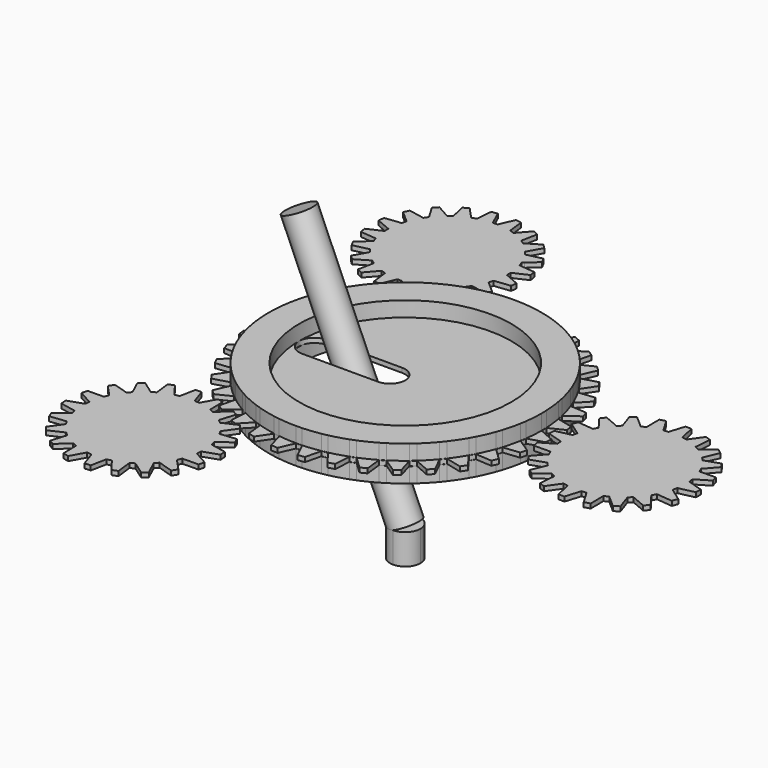
from build123d import *

# Parameters (mm, degrees)
F1_DEPTH  = 3
F2_DEPTH  = 3
F3_DEPTH  = 3
F4_DEPTH  = 3
F5_START  = 3.1
F5_DEPTH  = 10
F11_DEPTH = 20
F15_R     = 10


with BuildPart() as f1:
    # F0 (on Top) → F1 (new body)
    with BuildSketch(Plane.XY):
        with BuildLine():
            ThreePointArc((89.2300375236, -11.7473572998), (89.8073030915, -5.8862816307), (90, 0))
            Line((90, 0), (89.9143399424, 3.9257448629))
            ThreePointArc((89.9143399424, 3.9257448629), (89.46507044, 9.7980187367), (88.6326977711, 15.62833599))
            Line((88.6326977711, 15.62833599), (87.8666406408, 19.4795652544))
            ThreePointArc((87.8666406408, 19.4795652544), (86.4044868947, 25.1846112628), (84.5723358707, 30.7818128993))
            Line((84.5723358707, 30.7818128993), (83.149157926, 34.4415089129))
            ThreePointArc((83.149157926, 34.4415089129), (80.7185467379, 39.8059821197), (77.9422863406, 45))
            Line((77.9422863406, 45), (75.9052301232, 48.3569647512))
            ThreePointArc((75.9052301232, 48.3569647512), (72.5800143841, 53.2178683527), (68.9439998807, 57.8508848718))
            Line((68.9439998807, 57.8508848718), (66.3549603129, 60.8031186854))
            ThreePointArc((66.3549603129, 60.8031186854), (62.2361750204, 65.0127565854), (57.8508848718, 68.9439998807))
            Line((57.8508848718, 68.9439998807), (54.7885286108, 71.4018006262))
            ThreePointArc((54.7885286108, 71.4018006262), (50.0013209718, 74.8322651072), (45, 77.9422863406))
            Line((45, 77.9422863406), (41.5573751912, 79.830974986))
            ThreePointArc((41.5573751912, 79.830974986), (36.2472020873, 82.3780331208), (30.7818128993, 84.5723358707))
            Line((30.7818128993, 84.5723358707), (27.0635219554, 85.8345255673))
            ThreePointArc((27.0635219554, 85.8345255673), (21.3917303094, 87.4207862832), (15.62833599, 88.6326977711))
            Line((15.62833599, 88.6326977711), (11.7473572998, 89.2300375236))
            ThreePointArc((11.7473572998, 89.2300375236), (5.8862816307, 89.8073030915), (0, 90))
            Line((0, 90), (-3.9257448629, 89.9143399424))
            ThreePointArc((-3.9257448629, 89.9143399424), (-9.7980187367, 89.46507044), (-15.62833599, 88.6326977711))
            Line((-15.62833599, 88.6326977711), (-19.4795652544, 87.8666406408))
            ThreePointArc((-19.4795652544, 87.8666406408), (-25.1846112628, 86.4044868947), (-30.7818128993, 84.5723358707))
            Line((-30.7818128993, 84.5723358707), (-34.4415089129, 83.149157926))
            ThreePointArc((-34.4415089129, 83.149157926), (-39.8059821197, 80.7185467379), (-45, 77.9422863406))
            Line((-45, 77.9422863406), (-48.3569647512, 75.9052301232))
            ThreePointArc((-48.3569647512, 75.9052301232), (-53.2178683527, 72.5800143841), (-57.8508848718, 68.9439998807))
            Line((-57.8508848718, 68.9439998807), (-60.8031186854, 66.3549603129))
            ThreePointArc((-60.8031186854, 66.3549603129), (-65.0127565854, 62.2361750204), (-68.9439998807, 57.8508848718))
            Line((-68.9439998807, 57.8508848718), (-71.4018006262, 54.7885286108))
            ThreePointArc((-71.4018006262, 54.7885286108), (-74.8322651072, 50.0013209718), (-77.9422863406, 45))
            Line((-77.9422863406, 45), (-79.830974986, 41.5573751912))
            ThreePointArc((-79.830974986, 41.5573751912), (-82.3780331208, 36.2472020873), (-84.5723358707, 30.7818128993))
            Line((-84.5723358707, 30.7818128993), (-85.8345255673, 27.0635219554))
            ThreePointArc((-85.8345255673, 27.0635219554), (-87.4207862832, 21.3917303094), (-88.6326977711, 15.62833599))
            Line((-88.6326977711, 15.62833599), (-89.2300375236, 11.7473572998))
            ThreePointArc((-89.2300375236, 11.7473572998), (-89.8073030915, 5.8862816307), (-90, 0))
            Line((-90, 0), (-89.9143399424, -3.9257448629))
            ThreePointArc((-89.9143399424, -3.9257448629), (-89.46507044, -9.7980187367), (-88.6326977711, -15.62833599))
            Line((-88.6326977711, -15.62833599), (-87.8666406408, -19.4795652544))
            ThreePointArc((-87.8666406408, -19.4795652544), (-86.4044868947, -25.1846112628), (-84.5723358707, -30.7818128993))
            Line((-84.5723358707, -30.7818128993), (-83.149157926, -34.4415089129))
            ThreePointArc((-83.149157926, -34.4415089129), (-80.7185467379, -39.8059821197), (-77.9422863406, -45))
            Line((-77.9422863406, -45), (-75.9052301232, -48.3569647512))
            ThreePointArc((-75.9052301232, -48.3569647512), (-72.5800143841, -53.2178683527), (-68.9439998807, -57.8508848718))
            Line((-68.9439998807, -57.8508848718), (-66.3549603129, -60.8031186854))
            ThreePointArc((-66.3549603129, -60.8031186854), (-62.2361750204, -65.0127565854), (-57.8508848718, -68.9439998807))
            Line((-57.8508848718, -68.9439998807), (-54.7885286108, -71.4018006262))
            ThreePointArc((-54.7885286108, -71.4018006262), (-50.0013209718, -74.8322651072), (-45, -77.9422863406))
            Line((-45, -77.9422863406), (-41.5573751912, -79.830974986))
            ThreePointArc((-41.5573751912, -79.830974986), (-36.2472020873, -82.3780331208), (-30.7818128993, -84.5723358707))
            Line((-30.7818128993, -84.5723358707), (-27.0635219554, -85.8345255673))
            ThreePointArc((-27.0635219554, -85.8345255673), (-21.3917303094, -87.4207862832), (-15.62833599, -88.6326977711))
            Line((-15.62833599, -88.6326977711), (-11.7473572998, -89.2300375236))
            ThreePointArc((-11.7473572998, -89.2300375236), (-5.8862816307, -89.8073030915), (0, -90))
            Line((0, -90), (3.9257448629, -89.9143399424))
            ThreePointArc((3.9257448629, -89.9143399424), (9.7980187367, -89.46507044), (15.62833599, -88.6326977711))
            Line((15.62833599, -88.6326977711), (19.4795652544, -87.8666406408))
            ThreePointArc((19.4795652544, -87.8666406408), (25.1846112628, -86.4044868947), (30.7818128993, -84.5723358707))
            Line((30.7818128993, -84.5723358707), (34.4415089129, -83.149157926))
            ThreePointArc((34.4415089129, -83.149157926), (39.8059821197, -80.7185467379), (45, -77.9422863406))
            Line((45, -77.9422863406), (48.3569647512, -75.9052301232))
            ThreePointArc((48.3569647512, -75.9052301232), (53.2178683527, -72.5800143841), (57.8508848718, -68.9439998807))
            Line((57.8508848718, -68.9439998807), (60.8031186854, -66.3549603129))
            ThreePointArc((60.8031186854, -66.3549603129), (65.0127565854, -62.2361750204), (68.9439998807, -57.8508848718))
            Line((68.9439998807, -57.8508848718), (71.4018006262, -54.7885286108))
            ThreePointArc((71.4018006262, -54.7885286108), (74.8322651072, -50.0013209718), (77.9422863406, -45))
            Line((77.9422863406, -45), (79.830974986, -41.5573751912))
            ThreePointArc((79.830974986, -41.5573751912), (82.3780331208, -36.2472020873), (84.5723358707, -30.7818128993))
            Line((84.5723358707, -30.7818128993), (85.8345255673, -27.0635219554))
            ThreePointArc((85.8345255673, -27.0635219554), (87.4207862832, -21.3917303094), (88.6326977711, -15.62833599))
            Line((88.6326977711, -15.62833599), (89.2300375236, -11.7473572998))
        make_face()
        with BuildLine():
            ThreePointArc((-70, 0), (0, 70), (70, 0))
            ThreePointArc((70, 0), (0, -70), (-70, 0))
        make_face(mode=Mode.SUBTRACT)
        with BuildLine():
            ThreePointArc((-10, 10), (-2.9289321881, 7.0710678119), (0, 0))
            Line((0, 0), (70, 0))
            ThreePointArc((70, 0), (0, 70), (-70, 0))
            ThreePointArc((-70, 0), (-67.0710678119, 7.0710678119), (-60, 10))
            Line((-60, 10), (-35, 10))
            Line((-35, 10), (-10, 10))
        make_face()
        with BuildLine():
            Line((70, 0), (0, 0))
            ThreePointArc((0, 0), (-2.9289321881, -7.0710678119), (-10, -10))
            Line((-10, -10), (-35, -10))
            Line((-35, -10), (-60, -10))
            ThreePointArc((-60, -10), (-67.0710678119, -7.0710678119), (-70, 0))
            ThreePointArc((-70, 0), (0, -70), (70, 0))
        make_face()
        with BuildLine():
            Line((99.9048221582, -4.3619387365), (90, 0))
            ThreePointArc((90, 0), (89.8073030915, -5.8862816307), (89.2300375236, -11.7473572998))
            Line((89.2300375236, -11.7473572998), (99.6194698092, -8.7155742748))
            Line((99.6194698092, -8.7155742748), (99.9048221582, -4.3619387365))
        make_face()
        with BuildLine():
            ThreePointArc((-45, 77.9422863406), (-39.8059821197, 80.7185467379), (-34.4415089129, 83.149157926))
            Line((-34.4415089129, 83.149157926), (-42.2618261741, 90.6307787037))
            Line((-42.2618261741, 90.6307787037), (-46.1748613235, 88.7010833178))
            Line((-46.1748613235, 88.7010833178), (-45, 77.9422863406))
        make_face()
        with BuildLine():
            ThreePointArc((-57.8508848718, 68.9439998807), (-53.2178683527, 72.5800143841), (-48.3569647512, 75.9052301232))
            Line((-48.3569647512, 75.9052301232), (-57.3576436351, 81.9152044289))
            Line((-57.3576436351, 81.9152044289), (-60.8761429009, 79.3353340291))
            Line((-60.8761429009, 79.3353340291), (-57.8508848718, 68.9439998807))
        make_face()
        with BuildLine():
            ThreePointArc((-68.9439998807, 57.8508848718), (-65.0127565854, 62.2361750204), (-60.8031186854, 66.3549603129))
            Line((-60.8031186854, 66.3549603129), (-70.7106781187, 70.7106781187))
            Line((-70.7106781187, 70.7106781187), (-73.727733681, 67.5590207616))
            Line((-73.727733681, 67.5590207616), (-68.9439998807, 57.8508848718))
        make_face()
        with BuildLine():
            ThreePointArc((-77.9422863406, 45), (-74.8322651072, 50.0013209718), (-71.4018006262, 54.7885286108))
            Line((-71.4018006262, 54.7885286108), (-81.9152044289, 57.3576436351))
            Line((-81.9152044289, 57.3576436351), (-84.3391445813, 53.7299608347))
            Line((-84.3391445813, 53.7299608347), (-77.9422863406, 45))
        make_face()
        with BuildLine():
            ThreePointArc((-84.5723358707, 30.7818128993), (-82.3780331208, 36.2472020873), (-79.830974986, 41.5573751912))
            Line((-79.830974986, 41.5573751912), (-90.6307787037, 42.2618261741))
            Line((-90.6307787037, 42.2618261741), (-92.3879532511, 38.2683432365))
            Line((-92.3879532511, 38.2683432365), (-84.5723358707, 30.7818128993))
        make_face()
        with BuildLine():
            Line((-99.1444861374, -13.052619222), (-88.6326977711, -15.62833599))
            ThreePointArc((-88.6326977711, -15.62833599), (-89.46507044, -9.7980187367), (-89.9143399424, -3.9257448629))
            Line((-89.9143399424, -3.9257448629), (-99.6194698092, -8.7155742748))
            Line((-99.6194698092, -8.7155742748), (-99.1444861374, -13.052619222))
        make_face()
        with BuildLine():
            ThreePointArc((-88.6326977711, 15.62833599), (-87.4207862832, 21.3917303094), (-85.8345255673, 27.0635219554))
            Line((-85.8345255673, 27.0635219554), (-96.5925826289, 25.8819045103))
            Line((-96.5925826289, 25.8819045103), (-97.629600712, 21.6439613938))
            Line((-97.629600712, 21.6439613938), (-88.6326977711, 15.62833599))
        make_face()
        with BuildLine():
            ThreePointArc((-90, 0), (-89.8073030915, 5.8862816307), (-89.2300375236, 11.7473572998))
            Line((-89.2300375236, 11.7473572998), (-99.6194698092, 8.7155742748))
            Line((-99.6194698092, 8.7155742748), (-99.9048221582, 4.3619387365))
            Line((-99.9048221582, 4.3619387365), (-90, 0))
        make_face()
        with BuildLine():
            Line((-88.7010833178, -46.1748613235), (-77.9422863406, -45))
            ThreePointArc((-77.9422863406, -45), (-80.7185467379, -39.8059821197), (-83.149157926, -34.4415089129))
            Line((-83.149157926, -34.4415089129), (-90.6307787037, -42.2618261741))
            Line((-90.6307787037, -42.2618261741), (-88.7010833178, -46.1748613235))
        make_face()
        with BuildLine():
            Line((-79.3353340291, -60.8761429009), (-68.9439998807, -57.8508848718))
            ThreePointArc((-68.9439998807, -57.8508848718), (-72.5800143841, -53.2178683527), (-75.9052301232, -48.3569647512))
            Line((-75.9052301232, -48.3569647512), (-81.9152044289, -57.3576436351))
            Line((-81.9152044289, -57.3576436351), (-79.3353340291, -60.8761429009))
        make_face()
        with BuildLine():
            Line((-95.3716950748, -30.0705799504), (-84.5723358707, -30.7818128993))
            ThreePointArc((-84.5723358707, -30.7818128993), (-86.4044868947, -25.1846112628), (-87.8666406408, -19.4795652544))
            Line((-87.8666406408, -19.4795652544), (-96.5925826289, -25.8819045103))
            Line((-96.5925826289, -25.8819045103), (-95.3716950748, -30.0705799504))
        make_face()
        with BuildLine():
            Line((60.8761429009, -79.3353340291), (57.8508848718, -68.9439998807))
            ThreePointArc((57.8508848718, -68.9439998807), (53.2178683527, -72.5800143841), (48.3569647512, -75.9052301232))
            Line((48.3569647512, -75.9052301232), (57.3576436351, -81.9152044289))
            Line((57.3576436351, -81.9152044289), (60.8761429009, -79.3353340291))
        make_face()
        with BuildLine():
            Line((73.727733681, -67.5590207616), (68.9439998807, -57.8508848718))
            ThreePointArc((68.9439998807, -57.8508848718), (65.0127565854, -62.2361750204), (60.8031186854, -66.3549603129))
            Line((60.8031186854, -66.3549603129), (70.7106781187, -70.7106781187))
            Line((70.7106781187, -70.7106781187), (73.727733681, -67.5590207616))
        make_face()
        with BuildLine():
            Line((84.3391445813, -53.7299608347), (77.9422863406, -45))
            ThreePointArc((77.9422863406, -45), (74.8322651072, -50.0013209718), (71.4018006262, -54.7885286108))
            Line((71.4018006262, -54.7885286108), (81.9152044289, -57.3576436351))
            Line((81.9152044289, -57.3576436351), (84.3391445813, -53.7299608347))
        make_face()
        with BuildLine():
            Line((92.3879532511, -38.2683432365), (84.5723358707, -30.7818128993))
            ThreePointArc((84.5723358707, -30.7818128993), (82.3780331208, -36.2472020873), (79.830974986, -41.5573751912))
            Line((79.830974986, -41.5573751912), (90.6307787037, -42.2618261741))
            Line((90.6307787037, -42.2618261741), (92.3879532511, -38.2683432365))
        make_face()
        with BuildLine():
            Line((30.0705799504, -95.3716950748), (30.7818128993, -84.5723358707))
            ThreePointArc((30.7818128993, -84.5723358707), (25.1846112628, -86.4044868947), (19.4795652544, -87.8666406408))
            Line((19.4795652544, -87.8666406408), (25.8819045103, -96.5925826289))
            Line((25.8819045103, -96.5925826289), (30.0705799504, -95.3716950748))
        make_face()
        with BuildLine():
            Line((46.1748613235, -88.7010833178), (45, -77.9422863406))
            ThreePointArc((45, -77.9422863406), (39.8059821197, -80.7185467379), (34.4415089129, -83.149157926))
            Line((34.4415089129, -83.149157926), (42.2618261741, -90.6307787037))
            Line((42.2618261741, -90.6307787037), (46.1748613235, -88.7010833178))
        make_face()
        with BuildLine():
            Line((13.052619222, -99.1444861374), (15.62833599, -88.6326977711))
            ThreePointArc((15.62833599, -88.6326977711), (9.7980187367, -89.46507044), (3.9257448629, -89.9143399424))
            Line((3.9257448629, -89.9143399424), (8.7155742748, -99.6194698092))
            Line((8.7155742748, -99.6194698092), (13.052619222, -99.1444861374))
        make_face()
        with BuildLine():
            Line((-4.3619387365, -99.9048221582), (0, -90))
            ThreePointArc((0, -90), (-5.8862816307, -89.8073030915), (-11.7473572998, -89.2300375236))
            Line((-11.7473572998, -89.2300375236), (-8.7155742748, -99.6194698092))
            Line((-8.7155742748, -99.6194698092), (-4.3619387365, -99.9048221582))
        make_face()
        with BuildLine():
            Line((-21.6439613938, -97.629600712), (-15.62833599, -88.6326977711))
            ThreePointArc((-15.62833599, -88.6326977711), (-21.3917303094, -87.4207862832), (-27.0635219554, -85.8345255673))
            Line((-27.0635219554, -85.8345255673), (-25.8819045103, -96.5925826289))
            Line((-25.8819045103, -96.5925826289), (-21.6439613938, -97.629600712))
        make_face()
        with BuildLine():
            Line((-38.2683432365, -92.3879532511), (-30.7818128993, -84.5723358707))
            ThreePointArc((-30.7818128993, -84.5723358707), (-36.2472020873, -82.3780331208), (-41.5573751912, -79.830974986))
            Line((-41.5573751912, -79.830974986), (-42.2618261741, -90.6307787037))
            Line((-42.2618261741, -90.6307787037), (-38.2683432365, -92.3879532511))
        make_face()
        with BuildLine():
            Line((-53.7299608347, -84.3391445813), (-45, -77.9422863406))
            ThreePointArc((-45, -77.9422863406), (-50.0013209718, -74.8322651072), (-54.7885286108, -71.4018006262))
            Line((-54.7885286108, -71.4018006262), (-57.3576436351, -81.9152044289))
            Line((-57.3576436351, -81.9152044289), (-53.7299608347, -84.3391445813))
        make_face()
        with BuildLine():
            Line((-67.5590207616, -73.727733681), (-57.8508848718, -68.9439998807))
            ThreePointArc((-57.8508848718, -68.9439998807), (-62.2361750204, -65.0127565854), (-66.3549603129, -60.8031186854))
            Line((-66.3549603129, -60.8031186854), (-70.7106781187, -70.7106781187))
            Line((-70.7106781187, -70.7106781187), (-67.5590207616, -73.727733681))
        make_face()
        with BuildLine():
            Line((97.629600712, -21.6439613938), (88.6326977711, -15.62833599))
            ThreePointArc((88.6326977711, -15.62833599), (87.4207862832, -21.3917303094), (85.8345255673, -27.0635219554))
            Line((85.8345255673, -27.0635219554), (96.5925826289, -25.8819045103))
            Line((96.5925826289, -25.8819045103), (97.629600712, -21.6439613938))
        make_face()
        with BuildLine():
            ThreePointArc((88.6326977711, 15.62833599), (89.46507044, 9.7980187367), (89.9143399424, 3.9257448629))
            Line((89.9143399424, 3.9257448629), (99.6194698092, 8.7155742748))
            Line((99.6194698092, 8.7155742748), (99.1444861374, 13.052619222))
            Line((99.1444861374, 13.052619222), (88.6326977711, 15.62833599))
        make_face()
        with BuildLine():
            ThreePointArc((84.5723358707, 30.7818128993), (86.4044868947, 25.1846112628), (87.8666406408, 19.4795652544))
            Line((87.8666406408, 19.4795652544), (96.5925826289, 25.8819045103))
            Line((96.5925826289, 25.8819045103), (95.3716950748, 30.0705799504))
            Line((95.3716950748, 30.0705799504), (84.5723358707, 30.7818128993))
        make_face()
        with BuildLine():
            ThreePointArc((77.9422863406, 45), (80.7185467379, 39.8059821197), (83.149157926, 34.4415089129))
            Line((83.149157926, 34.4415089129), (90.6307787037, 42.2618261741))
            Line((90.6307787037, 42.2618261741), (88.7010833178, 46.1748613235))
            Line((88.7010833178, 46.1748613235), (77.9422863406, 45))
        make_face()
        with BuildLine():
            ThreePointArc((68.9439998807, 57.8508848718), (72.5800143841, 53.2178683527), (75.9052301232, 48.3569647512))
            Line((75.9052301232, 48.3569647512), (81.9152044289, 57.3576436351))
            Line((81.9152044289, 57.3576436351), (79.3353340291, 60.8761429009))
            Line((79.3353340291, 60.8761429009), (68.9439998807, 57.8508848718))
        make_face()
        with BuildLine():
            ThreePointArc((57.8508848718, 68.9439998807), (62.2361750204, 65.0127565854), (66.3549603129, 60.8031186854))
            Line((66.3549603129, 60.8031186854), (70.7106781187, 70.7106781187))
            Line((70.7106781187, 70.7106781187), (67.5590207616, 73.727733681))
            Line((67.5590207616, 73.727733681), (57.8508848718, 68.9439998807))
        make_face()
        with BuildLine():
            ThreePointArc((45, 77.9422863406), (50.0013209718, 74.8322651072), (54.7885286108, 71.4018006262))
            Line((54.7885286108, 71.4018006262), (57.3576436351, 81.9152044289))
            Line((57.3576436351, 81.9152044289), (53.7299608347, 84.3391445813))
            Line((53.7299608347, 84.3391445813), (45, 77.9422863406))
        make_face()
        with BuildLine():
            ThreePointArc((30.7818128993, 84.5723358707), (36.2472020873, 82.3780331208), (41.5573751912, 79.830974986))
            Line((41.5573751912, 79.830974986), (42.2618261741, 90.6307787037))
            Line((42.2618261741, 90.6307787037), (38.2683432365, 92.3879532511))
            Line((38.2683432365, 92.3879532511), (30.7818128993, 84.5723358707))
        make_face()
        with BuildLine():
            ThreePointArc((-30.7818128993, 84.5723358707), (-25.1846112628, 86.4044868947), (-19.4795652544, 87.8666406408))
            Line((-19.4795652544, 87.8666406408), (-25.8819045103, 96.5925826289))
            Line((-25.8819045103, 96.5925826289), (-30.0705799504, 95.3716950748))
            Line((-30.0705799504, 95.3716950748), (-30.7818128993, 84.5723358707))
        make_face()
        with BuildLine():
            ThreePointArc((-15.62833599, 88.6326977711), (-9.7980187367, 89.46507044), (-3.9257448629, 89.9143399424))
            Line((-3.9257448629, 89.9143399424), (-8.7155742748, 99.6194698092))
            Line((-8.7155742748, 99.6194698092), (-13.052619222, 99.1444861374))
            Line((-13.052619222, 99.1444861374), (-15.62833599, 88.6326977711))
        make_face()
        with BuildLine():
            ThreePointArc((0, 90), (5.8862816307, 89.8073030915), (11.7473572998, 89.2300375236))
            Line((11.7473572998, 89.2300375236), (8.7155742748, 99.6194698092))
            Line((8.7155742748, 99.6194698092), (4.3619387365, 99.9048221582))
            Line((4.3619387365, 99.9048221582), (0, 90))
        make_face()
        with BuildLine():
            ThreePointArc((15.62833599, 88.6326977711), (21.3917303094, 87.4207862832), (27.0635219554, 85.8345255673))
            Line((27.0635219554, 85.8345255673), (25.8819045103, 96.5925826289))
            Line((25.8819045103, 96.5925826289), (21.6439613938, 97.629600712))
            Line((21.6439613938, 97.629600712), (15.62833599, 88.6326977711))
        make_face()
        with BuildLine():
            ThreePointArc((-84.5723358707, -30.7818128993), (-83.8807082355, -32.6194234455), (-83.149157926, -34.4415089129))
            Line((-83.149157926, -34.4415089129), (-84.5723358707, -30.7818128993))
        make_face()
        with BuildLine():
            ThreePointArc((-90, 0), (-89.9785824372, -1.9633396531), (-89.9143399424, -3.9257448629))
            Line((-89.9143399424, -3.9257448629), (-90, 0))
        make_face()
        with BuildLine():
            Line((-85.8345255673, 27.0635219554), (-84.5723358707, 30.7818128993))
            ThreePointArc((-84.5723358707, 30.7818128993), (-85.2237116546, 28.9295518773), (-85.8345255673, 27.0635219554))
        make_face()
        with BuildLine():
            ThreePointArc((-68.9439998807, -57.8508848718), (-67.6655826731, -59.341123359), (-66.3549603129, -60.8031186854))
            Line((-66.3549603129, -60.8031186854), (-68.9439998807, -57.8508848718))
        make_face()
        with BuildLine():
            Line((-89.2300375236, 11.7473572998), (-88.6326977711, 15.62833599))
            ThreePointArc((-88.6326977711, 15.62833599), (-88.9525359421, 13.6911047571), (-89.2300375236, 11.7473572998))
        make_face()
        with BuildLine():
            ThreePointArc((-88.6326977711, -15.62833599), (-88.2706752363, -17.5581289815), (-87.8666406408, -19.4795652544))
            Line((-87.8666406408, -19.4795652544), (-88.6326977711, -15.62833599))
        make_face()
        with BuildLine():
            ThreePointArc((-77.9422863406, -45), (-76.9420683606, -46.6895932344), (-75.9052301232, -48.3569647512))
            Line((-75.9052301232, -48.3569647512), (-77.9422863406, -45))
        make_face()
        with BuildLine():
            Line((-79.830974986, 41.5573751912), (-77.9422863406, 45))
            ThreePointArc((-77.9422863406, 45), (-78.9054080137, 43.2889892027), (-79.830974986, 41.5573751912))
        make_face()
        with BuildLine():
            ThreePointArc((77.9422863406, -45), (78.9054080137, -43.2889892027), (79.830974986, -41.5573751912))
            Line((79.830974986, -41.5573751912), (77.9422863406, -45))
        make_face()
        with BuildLine():
            ThreePointArc((84.5723358707, -30.7818128993), (85.2237116546, -28.9295518773), (85.8345255673, -27.0635219554))
            Line((85.8345255673, -27.0635219554), (84.5723358707, -30.7818128993))
        make_face()
        with BuildLine():
            ThreePointArc((45, -77.9422863406), (46.6895932344, -76.9420683606), (48.3569647512, -75.9052301232))
            Line((48.3569647512, -75.9052301232), (45, -77.9422863406))
        make_face()
        with BuildLine():
            ThreePointArc((68.9439998807, -57.8508848718), (70.1896034784, -56.3331124966), (71.4018006262, -54.7885286108))
            Line((71.4018006262, -54.7885286108), (68.9439998807, -57.8508848718))
        make_face()
        with BuildLine():
            ThreePointArc((30.7818128993, -84.5723358707), (32.6194234455, -83.8807082355), (34.4415089129, -83.149157926))
            Line((34.4415089129, -83.149157926), (30.7818128993, -84.5723358707))
        make_face()
        with BuildLine():
            ThreePointArc((15.62833599, -88.6326977711), (17.5581289815, -88.2706752363), (19.4795652544, -87.8666406408))
            Line((19.4795652544, -87.8666406408), (15.62833599, -88.6326977711))
        make_face()
        with BuildLine():
            ThreePointArc((57.8508848718, -68.9439998807), (59.341123359, -67.6655826731), (60.8031186854, -66.3549603129))
            Line((60.8031186854, -66.3549603129), (57.8508848718, -68.9439998807))
        make_face()
    extrude(amount=F1_DEPTH)


with BuildPart() as f2:
    # F0 (on Top) → F2 (new body)
    with BuildSketch(Plane.XY):
        with BuildLine():
            ThreePointArc((139.4889503814, 39.59586748), (143.6156290334, 19.9887742833), (145, 0))
            ThreePointArc((145, 0), (143.5126118837, -20.7154587281), (139.0809623405, -41.0059253577))
            Line((139.0809623405, -41.0059253577), (141.0770452136, -49.8458666867))
            Line((141.0770452136, -49.8458666867), (145, -50))
            Line((145, -50), (148.1383638291, -39.8766933493))
            Line((148.1383638291, -39.8766933493), (151.2573786016, -39.5075336238))
            Line((151.2573786016, -39.5075336238), (156.6722681928, -48.6184960199))
            Line((156.6722681928, -48.6184960199), (160.4508497187, -47.5528258148))
            Line((160.4508497187, -47.5528258148), (160.3073372946, -36.9551813005))
            Line((160.3073372946, -36.9551813005), (163.1596199896, -35.6402609675))
            Line((163.1596199896, -35.6402609675), (171.1249282358, -42.6320082177))
            Line((171.1249282358, -42.6320082177), (174.3892626146, -40.4508497187))
            Line((174.3892626146, -40.4508497187), (170.9779219332, -30.416238624))
            Line((170.9779219332, -30.416238624), (173.2842712475, -28.2842712475))
            Line((173.2842712475, -28.2842712475), (183.02029828, -32.4724024165))
            Line((183.02029828, -32.4724024165), (185.4508497187, -29.3892626146))
            Line((185.4508497187, -29.3892626146), (179.1056065742, -20.8999425886))
            Line((179.1056065742, -20.8999425886), (180.6402609675, -18.1596199896))
            Line((180.6402609675, -18.1596199896), (191.1939766256, -19.1341716183))
            Line((191.1939766256, -19.1341716183), (192.5528258148, -15.4508497187))
            Line((192.5528258148, -15.4508497187), (183.8947968159, -9.3378145542))
            Line((183.8947968159, -9.3378145542), (184.5075336238, -6.2573786016))
            Line((184.5075336238, -6.2573786016), (194.8458666867, -3.9229547864))
            Line((194.8458666867, -3.9229547864), (195, 0))
            Line((195, 0), (184.8766933493, 3.1383638291))
            Line((184.8766933493, 3.1383638291), (184.5075336238, 6.2573786016))
            Line((184.5075336238, 6.2573786016), (193.6184960199, 11.6722681928))
            Line((193.6184960199, 11.6722681928), (192.5528258148, 15.4508497187))
            Line((192.5528258148, 15.4508497187), (181.9551813005, 15.3073372946))
            Line((181.9551813005, 15.3073372946), (180.6402609675, 18.1596199896))
            Line((180.6402609675, 18.1596199896), (187.6320082177, 26.1249282358))
            Line((187.6320082177, 26.1249282358), (185.4508497187, 29.3892626146))
            Line((185.4508497187, 29.3892626146), (175.416238624, 25.9779219332))
            Line((175.416238624, 25.9779219332), (173.2842712475, 28.2842712475))
            Line((173.2842712475, 28.2842712475), (177.4724024165, 38.02029828))
            Line((177.4724024165, 38.02029828), (174.3892626146, 40.4508497187))
            Line((174.3892626146, 40.4508497187), (165.8999425886, 34.1056065742))
            Line((165.8999425886, 34.1056065742), (163.1596199896, 35.6402609675))
            Line((163.1596199896, 35.6402609675), (164.1341716183, 46.1939766256))
            Line((164.1341716183, 46.1939766256), (160.4508497187, 47.5528258148))
            Line((160.4508497187, 47.5528258148), (154.3378145542, 38.8947968159))
            Line((154.3378145542, 38.8947968159), (151.2573786016, 39.5075336238))
            Line((151.2573786016, 39.5075336238), (148.9229547864, 49.8458666867))
            Line((148.9229547864, 49.8458666867), (145, 50))
            Line((145, 50), (141.8616361709, 39.8766933493))
            Line((141.8616361709, 39.8766933493), (139.4889503814, 39.59586748))
        make_face()
        with BuildLine():
            Line((95.1541333133, 3.9229547864), (95, 0))
            Line((95, 0), (100, 0))
            Line((100, 0), (145, 0))
            ThreePointArc((145, 0), (143.6156290334, 19.9887742833), (139.4889503814, 39.59586748))
            Line((139.4889503814, 39.59586748), (138.7426213984, 39.5075336238))
            Line((138.7426213984, 39.5075336238), (133.3277318072, 48.6184960199))
            Line((133.3277318072, 48.6184960199), (129.5491502813, 47.5528258148))
            Line((129.5491502813, 47.5528258148), (129.6926627054, 36.9551813005))
            Line((129.6926627054, 36.9551813005), (126.8403800104, 35.6402609675))
            Line((126.8403800104, 35.6402609675), (118.8750717642, 42.6320082177))
            Line((118.8750717642, 42.6320082177), (115.6107373854, 40.4508497187))
            Line((115.6107373854, 40.4508497187), (119.0220780668, 30.416238624))
            Line((119.0220780668, 30.416238624), (116.7157287525, 28.2842712475))
            Line((116.7157287525, 28.2842712475), (106.97970172, 32.4724024165))
            Line((106.97970172, 32.4724024165), (104.5491502813, 29.3892626146))
            Line((104.5491502813, 29.3892626146), (110.8943934258, 20.8999425886))
            Line((110.8943934258, 20.8999425886), (109.3597390325, 18.1596199896))
            Line((109.3597390325, 18.1596199896), (98.8060233744, 19.1341716183))
            Line((98.8060233744, 19.1341716183), (97.4471741852, 15.4508497187))
            Line((97.4471741852, 15.4508497187), (106.1052031841, 9.3378145542))
            Line((106.1052031841, 9.3378145542), (105.4924663762, 6.2573786016))
            Line((105.4924663762, 6.2573786016), (95.1541333133, 3.9229547864))
        make_face()
        with BuildLine():
            Line((100, 0), (95, 0))
            Line((95, 0), (105.1233066507, -3.1383638291))
            Line((105.1233066507, -3.1383638291), (105.4924663762, -6.2573786016))
            Line((105.4924663762, -6.2573786016), (96.3815039801, -11.6722681928))
            Line((96.3815039801, -11.6722681928), (97.4471741852, -15.4508497187))
            Line((97.4471741852, -15.4508497187), (108.0448186995, -15.3073372946))
            Line((108.0448186995, -15.3073372946), (109.3597390325, -18.1596199896))
            Line((109.3597390325, -18.1596199896), (102.3679917823, -26.1249282358))
            Line((102.3679917823, -26.1249282358), (104.5491502813, -29.3892626146))
            Line((104.5491502813, -29.3892626146), (114.583761376, -25.9779219332))
            Line((114.583761376, -25.9779219332), (116.7157287525, -28.2842712475))
            Line((116.7157287525, -28.2842712475), (112.5275975835, -38.02029828))
            Line((112.5275975835, -38.02029828), (115.6107373854, -40.4508497187))
            Line((115.6107373854, -40.4508497187), (124.1000574114, -34.1056065742))
            Line((124.1000574114, -34.1056065742), (126.8403800104, -35.6402609675))
            Line((126.8403800104, -35.6402609675), (125.8658283817, -46.1939766256))
            Line((125.8658283817, -46.1939766256), (129.5491502813, -47.5528258148))
            Line((129.5491502813, -47.5528258148), (135.6621854458, -38.8947968159))
            Line((135.6621854458, -38.8947968159), (138.7426213984, -39.5075336238))
            Line((138.7426213984, -39.5075336238), (139.0809623405, -41.0059253577))
            ThreePointArc((139.0809623405, -41.0059253577), (143.5126118837, -20.7154587281), (145, 0))
            Line((145, 0), (100, 0))
        make_face()
    extrude(amount=F2_DEPTH)


with BuildPart() as f3:
    # F0 (on Top) → F3 (new body)
    with BuildSketch(Plane.XY):
        with BuildLine():
            Line((-35.1567829401, 139.9084015306), (-34.0283081048, 140.9506092485))
            ThreePointArc((-34.0283081048, 140.9506092485), (-71.8634538015, 125.9390487804), (-104.0355023133, 101.0030408375))
            Line((-104.0355023133, 101.0030408375), (-103.5858384583, 100.4008679068))
            Line((-103.5858384583, 100.4008679068), (-108.7687185506, 91.1559547641))
            Line((-108.7687185506, 91.1559547641), (-105.9565303179, 88.4164422749))
            Line((-105.9565303179, 88.4164422749), (-96.8504571603, 93.8395499371))
            Line((-96.8504571603, 93.8395499371), (-94.2855614006, 92.0268608309))
            Line((-94.2855614006, 92.0268608309), (-96.357938013, 81.6328279156))
            Line((-96.357938013, 81.6328279156), (-92.8368321538, 79.8964106666))
            Line((-92.8368321538, 79.8964106666), (-85.8522743694, 87.8680239051))
            Line((-85.8522743694, 87.8680239051), (-82.8527618041, 86.9366504972))
            Line((-82.8527618041, 86.9366504972), (-81.6117762746, 76.4109381705))
            Line((-81.6117762746, 76.4109381705), (-77.7264231634, 75.8475887803))
            Line((-77.7264231634, 75.8475887803), (-73.5470779323, 85.5873905497))
            Line((-73.5470779323, 85.5873905497), (-70.4065617503, 85.6285021586))
            Line((-70.4065617503, 85.6285021586), (-65.973690389, 76.0014404801))
            Line((-65.973690389, 76.0014404801), (-62.1044154591, 76.6663035121))
            Line((-62.1044154591, 76.6663035121), (-61.1393862118, 87.220894154))
            Line((-61.1393862118, 87.220894154), (-58.1652820182, 88.2304664889))
            Line((-58.1652820182, 88.2304664889), (-50.9744451596, 80.4444193313))
            Line((-50.9744451596, 80.4444193313), (-47.5, 82.2724133595))
            Line((-47.5, 82.2724133595), (-49.843750523, 92.6086360039))
            Line((-49.843750523, 92.6086360039), (-47.327184358, 94.4878450905))
            Line((-47.327184358, 94.4878450905), (-38.0822712153, 89.3049649981))
            Line((-38.0822712153, 89.3049649981), (-35.3427587261, 92.1171532308))
            Line((-35.3427587261, 92.1171532308), (-40.7658663884, 101.2232263884))
            Line((-40.7658663884, 101.2232263884), (-38.9531772822, 103.7881221481))
            Line((-38.9531772822, 103.7881221481), (-28.5591443669, 101.7157455358))
            Line((-28.5591443669, 101.7157455358), (-26.8227271179, 105.236851395))
            Line((-26.8227271179, 105.236851395), (-34.7943403563, 112.2214091794))
            Line((-34.7943403563, 112.2214091794), (-33.8629669484, 115.2209217446))
            Line((-33.8629669484, 115.2209217446), (-23.3372546218, 116.4619072741))
            Line((-23.3372546218, 116.4619072741), (-22.7739052316, 120.3472603854))
            Line((-22.7739052316, 120.3472603854), (-32.513707001, 124.5266056164))
            Line((-32.513707001, 124.5266056164), (-32.5548186098, 127.6671217985))
            Line((-32.5548186098, 127.6671217985), (-22.9277569313, 132.0999931597))
            Line((-22.9277569313, 132.0999931597), (-23.5926199633, 135.9692680896))
            Line((-23.5926199633, 135.9692680896), (-34.1472106053, 136.9342973369))
            Line((-34.1472106053, 136.9342973369), (-35.1567829401, 139.9084015306))
        make_face()
        with BuildLine():
            ThreePointArc((-104.0355023133, 101.0030408375), (-71.8634538015, 125.9390487804), (-34.0283081048, 140.9506092485))
            Line((-34.0283081048, 140.9506092485), (-27.3707357825, 147.0992383892))
            Line((-27.3707357825, 147.0992383892), (-29.1987298108, 150.5736835487))
            Line((-29.1987298108, 150.5736835487), (-39.5349524551, 148.2299330257))
            Line((-39.5349524551, 148.2299330257), (-41.4141615417, 150.7464991907))
            Line((-41.4141615417, 150.7464991907), (-36.2312814494, 159.9914123334))
            Line((-36.2312814494, 159.9914123334), (-39.0434696821, 162.7309248226))
            Line((-39.0434696821, 162.7309248226), (-48.1495428397, 157.3078171604))
            Line((-48.1495428397, 157.3078171604), (-50.7144385994, 159.1205062666))
            Line((-50.7144385994, 159.1205062666), (-48.642061987, 169.5145391818))
            Line((-48.642061987, 169.5145391818), (-52.1631678462, 171.2509564309))
            Line((-52.1631678462, 171.2509564309), (-59.1477256306, 163.2793431924))
            Line((-59.1477256306, 163.2793431924), (-62.1472381959, 164.2107166003))
            Line((-62.1472381959, 164.2107166003), (-63.3882237254, 174.7364289269))
            Line((-63.3882237254, 174.7364289269), (-67.2735768366, 175.2997783172))
            Line((-67.2735768366, 175.2997783172), (-71.4529220677, 165.5599765478))
            Line((-71.4529220677, 165.5599765478), (-74.5934382497, 165.5188649389))
            Line((-74.5934382497, 165.5188649389), (-79.026309611, 175.1459266174))
            Line((-79.026309611, 175.1459266174), (-82.8955845409, 174.4810635854))
            Line((-82.8955845409, 174.4810635854), (-83.8606137882, 163.9264729435))
            Line((-83.8606137882, 163.9264729435), (-86.8347179818, 162.9169006086))
            Line((-86.8347179818, 162.9169006086), (-94.0255548404, 170.7029477662))
            Line((-94.0255548404, 170.7029477662), (-97.5, 168.874953738))
            Line((-97.5, 168.874953738), (-95.156249477, 158.5387310936))
            Line((-95.156249477, 158.5387310936), (-97.672815642, 156.659522007))
            Line((-97.672815642, 156.659522007), (-106.9177287847, 161.8424020994))
            Line((-106.9177287847, 161.8424020994), (-109.6572412739, 159.0302138667))
            Line((-109.6572412739, 159.0302138667), (-104.2341336116, 149.9241407091))
            Line((-104.2341336116, 149.9241407091), (-106.0468227178, 147.3592449493))
            Line((-106.0468227178, 147.3592449493), (-116.4408556331, 149.4316215617))
            Line((-116.4408556331, 149.4316215617), (-118.1772728821, 145.9105157025))
            Line((-118.1772728821, 145.9105157025), (-110.2056596437, 138.9259579181))
            Line((-110.2056596437, 138.9259579181), (-111.1370330516, 135.9264453528))
            Line((-111.1370330516, 135.9264453528), (-121.6627453782, 134.6854598234))
            Line((-121.6627453782, 134.6854598234), (-122.2260947684, 130.8001067121))
            Line((-122.2260947684, 130.8001067121), (-112.486292999, 126.6207614811))
            Line((-112.486292999, 126.6207614811), (-112.4451813902, 123.480245299))
            Line((-112.4451813902, 123.480245299), (-122.0722430687, 119.0473739377))
            Line((-122.0722430687, 119.0473739377), (-121.4073800367, 115.1780990079))
            Line((-121.4073800367, 115.1780990079), (-110.8527893947, 114.2130697606))
            Line((-110.8527893947, 114.2130697606), (-109.8432170599, 111.2389655669))
            Line((-109.8432170599, 111.2389655669), (-117.6292642175, 104.0481287083))
            Line((-117.6292642175, 104.0481287083), (-115.8012701892, 100.5736835487))
            Line((-115.8012701892, 100.5736835487), (-105.4650475449, 102.9174340718))
            Line((-105.4650475449, 102.9174340718), (-104.0355023133, 101.0030408375))
        make_face()
    extrude(amount=F3_DEPTH)


with BuildPart() as f4:
    # F0 (on Top) → F4 (new body)
    with BuildSketch(Plane.XY):
        with BuildLine():
            ThreePointArc((-105.0526542357, -99.9446838908), (-73.1346886716, -125.205100986), (-35.4534480681, -140.5989083175))
            Line((-35.4534480681, -140.5989083175), (-35.1567829401, -139.9084015306))
            Line((-35.1567829401, -139.9084015306), (-24.5590132566, -139.7744507839))
            Line((-24.5590132566, -139.7744507839), (-23.5926199633, -135.9692680896))
            Line((-23.5926199633, -135.9692680896), (-32.842205545, -130.7947312375))
            Line((-32.842205545, -130.7947312375), (-32.5548186098, -127.6671217985))
            Line((-32.5548186098, -127.6671217985), (-22.5171337512, -124.2648361333))
            Line((-22.5171337512, -124.2648361333), (-22.7739052316, -120.3472603854))
            Line((-22.7739052316, -120.3472603854), (-33.1698036974, -118.2842625291))
            Line((-33.1698036974, -118.2842625291), (-33.8629669484, -115.2209217446))
            Line((-33.8629669484, -115.2209217446), (-25.3679254454, -108.8833405871))
            Line((-25.3679254454, -108.8833405871), (-26.8227271179, -105.236851395))
            Line((-26.8227271179, -105.236851395), (-37.3473154935, -106.4873331384))
            Line((-37.3473154935, -106.4873331384), (-38.9531772822, -103.7881221481))
            Line((-38.9531772822, -103.7881221481), (-32.8323329854, -95.1356120983))
            Line((-32.8323329854, -95.1356120983), (-35.3427587261, -92.1171532308))
            Line((-35.3427587261, -92.1171532308), (-44.9658169722, -96.5587087083))
            Line((-44.9658169722, -96.5587087083), (-47.327184358, -94.4878450905))
            Line((-47.327184358, -94.4878450905), (-44.1796881538, -84.3673741176))
            Line((-44.1796881538, -84.3673741176), (-47.5, -82.2724133595))
            Line((-47.5, -82.2724133595), (-55.2795561277, -89.4702721747))
            Line((-55.2795561277, -89.4702721747), (-58.1652820182, -88.2304664889))
            Line((-58.1652820182, -88.2304664889), (-58.2992327648, -77.6326968053))
            Line((-58.2992327648, -77.6326968053), (-62.1044154591, -76.6663035121))
            Line((-62.1044154591, -76.6663035121), (-67.2789523112, -85.9158890938))
            Line((-67.2789523112, -85.9158890938), (-70.4065617503, -85.6285021586))
            Line((-70.4065617503, -85.6285021586), (-73.8088474154, -75.5908173))
            Line((-73.8088474154, -75.5908173), (-77.7264231634, -75.8475887803))
            Line((-77.7264231634, -75.8475887803), (-79.7894210197, -86.2434872462))
            Line((-79.7894210197, -86.2434872462), (-82.8527618041, -86.9366504972))
            Line((-82.8527618041, -86.9366504972), (-89.1903429617, -78.4416089941))
            Line((-89.1903429617, -78.4416089941), (-92.8368321538, -79.8964106666))
            Line((-92.8368321538, -79.8964106666), (-91.5863504104, -90.4209990423))
            Line((-91.5863504104, -90.4209990423), (-94.2855614006, -92.0268608309))
            Line((-94.2855614006, -92.0268608309), (-102.9380714504, -85.9060165342))
            Line((-102.9380714504, -85.9060165342), (-105.9565303179, -88.4164422749))
            Line((-105.9565303179, -88.4164422749), (-101.5149748405, -98.039500521))
            Line((-101.5149748405, -98.039500521), (-103.5858384583, -100.4008679068))
            Line((-103.5858384583, -100.4008679068), (-105.0526542357, -99.9446838908))
        make_face()
        with BuildLine():
            Line((-36.396588626, -142.7941274211), (-35.4534480681, -140.5989083175))
            ThreePointArc((-35.4534480681, -140.5989083175), (-73.1346886716, -125.205100986), (-105.0526542357, -99.9446838908))
            Line((-105.0526542357, -99.9446838908), (-113.7063094311, -97.2533717025))
            Line((-113.7063094311, -97.2533717025), (-115.8012701892, -100.5736835487))
            Line((-115.8012701892, -100.5736835487), (-108.603411374, -108.3532396764))
            Line((-108.603411374, -108.3532396764), (-109.8432170599, -111.2389655669))
            Line((-109.8432170599, -111.2389655669), (-120.4409867434, -111.3729163135))
            Line((-120.4409867434, -111.3729163135), (-121.4073800367, -115.1780990079))
            Line((-121.4073800367, -115.1780990079), (-112.157794455, -120.3526358599))
            Line((-112.157794455, -120.3526358599), (-112.4451813902, -123.480245299))
            Line((-112.4451813902, -123.480245299), (-122.4828662488, -126.8825309641))
            Line((-122.4828662488, -126.8825309641), (-122.2260947684, -130.8001067121))
            Line((-122.2260947684, -130.8001067121), (-111.8301963026, -132.8631045684))
            Line((-111.8301963026, -132.8631045684), (-111.1370330516, -135.9264453528))
            Line((-111.1370330516, -135.9264453528), (-119.6320745546, -142.2640265104))
            Line((-119.6320745546, -142.2640265104), (-118.1772728821, -145.9105157025))
            Line((-118.1772728821, -145.9105157025), (-107.6526845065, -144.6600339591))
            Line((-107.6526845065, -144.6600339591), (-106.0468227178, -147.3592449493))
            Line((-106.0468227178, -147.3592449493), (-112.1676670146, -156.0117549992))
            Line((-112.1676670146, -156.0117549992), (-109.6572412739, -159.0302138667))
            Line((-109.6572412739, -159.0302138667), (-100.0341830278, -154.5886583892))
            Line((-100.0341830278, -154.5886583892), (-97.672815642, -156.659522007))
            Line((-97.672815642, -156.659522007), (-100.8203118462, -166.7799929798))
            Line((-100.8203118462, -166.7799929798), (-97.5, -168.874953738))
            Line((-97.5, -168.874953738), (-89.7204438723, -161.6770949227))
            Line((-89.7204438723, -161.6770949227), (-86.8347179818, -162.9169006086))
            Line((-86.8347179818, -162.9169006086), (-86.7007672352, -173.5146702922))
            Line((-86.7007672352, -173.5146702922), (-82.8955845409, -174.4810635854))
            Line((-82.8955845409, -174.4810635854), (-77.7210476888, -165.2314780037))
            Line((-77.7210476888, -165.2314780037), (-74.5934382497, -165.5188649389))
            Line((-74.5934382497, -165.5188649389), (-71.1911525846, -175.5565497975))
            Line((-71.1911525846, -175.5565497975), (-67.2735768366, -175.2997783172))
            Line((-67.2735768366, -175.2997783172), (-65.2105789803, -164.9038798513))
            Line((-65.2105789803, -164.9038798513), (-62.1472381959, -164.2107166003))
            Line((-62.1472381959, -164.2107166003), (-55.8096570383, -172.7057581034))
            Line((-55.8096570383, -172.7057581034), (-52.1631678462, -171.2509564309))
            Line((-52.1631678462, -171.2509564309), (-53.4136495896, -160.7263680552))
            Line((-53.4136495896, -160.7263680552), (-50.7144385994, -159.1205062666))
            Line((-50.7144385994, -159.1205062666), (-42.0619285496, -165.2413505633))
            Line((-42.0619285496, -165.2413505633), (-39.0434696821, -162.7309248226))
            Line((-39.0434696821, -162.7309248226), (-43.4850251595, -153.1078665765))
            Line((-43.4850251595, -153.1078665765), (-41.4141615417, -150.7464991907))
            Line((-41.4141615417, -150.7464991907), (-31.2936905689, -153.893995395))
            Line((-31.2936905689, -153.893995395), (-29.1987298108, -150.5736835487))
            Line((-29.1987298108, -150.5736835487), (-36.396588626, -142.7941274211))
        make_face()
    extrude(amount=F4_DEPTH)


with BuildPart() as f5:
    # F0 (on Top) → F5 (new body)
    with BuildSketch(Plane.XY.offset(F5_START)):
        with BuildLine():
            ThreePointArc((89.2300375236, -11.7473572998), (89.8073030915, -5.8862816307), (90, 0))
            Line((90, 0), (89.9143399424, 3.9257448629))
            ThreePointArc((89.9143399424, 3.9257448629), (89.46507044, 9.7980187367), (88.6326977711, 15.62833599))
            Line((88.6326977711, 15.62833599), (87.8666406408, 19.4795652544))
            ThreePointArc((87.8666406408, 19.4795652544), (86.4044868947, 25.1846112628), (84.5723358707, 30.7818128993))
            Line((84.5723358707, 30.7818128993), (83.149157926, 34.4415089129))
            ThreePointArc((83.149157926, 34.4415089129), (80.7185467379, 39.8059821197), (77.9422863406, 45))
            Line((77.9422863406, 45), (75.9052301232, 48.3569647512))
            ThreePointArc((75.9052301232, 48.3569647512), (72.5800143841, 53.2178683527), (68.9439998807, 57.8508848718))
            Line((68.9439998807, 57.8508848718), (66.3549603129, 60.8031186854))
            ThreePointArc((66.3549603129, 60.8031186854), (62.2361750204, 65.0127565854), (57.8508848718, 68.9439998807))
            Line((57.8508848718, 68.9439998807), (54.7885286108, 71.4018006262))
            ThreePointArc((54.7885286108, 71.4018006262), (50.0013209718, 74.8322651072), (45, 77.9422863406))
            Line((45, 77.9422863406), (41.5573751912, 79.830974986))
            ThreePointArc((41.5573751912, 79.830974986), (36.2472020873, 82.3780331208), (30.7818128993, 84.5723358707))
            Line((30.7818128993, 84.5723358707), (27.0635219554, 85.8345255673))
            ThreePointArc((27.0635219554, 85.8345255673), (21.3917303094, 87.4207862832), (15.62833599, 88.6326977711))
            Line((15.62833599, 88.6326977711), (11.7473572998, 89.2300375236))
            ThreePointArc((11.7473572998, 89.2300375236), (5.8862816307, 89.8073030915), (0, 90))
            Line((0, 90), (-3.9257448629, 89.9143399424))
            ThreePointArc((-3.9257448629, 89.9143399424), (-9.7980187367, 89.46507044), (-15.62833599, 88.6326977711))
            Line((-15.62833599, 88.6326977711), (-19.4795652544, 87.8666406408))
            ThreePointArc((-19.4795652544, 87.8666406408), (-25.1846112628, 86.4044868947), (-30.7818128993, 84.5723358707))
            Line((-30.7818128993, 84.5723358707), (-34.4415089129, 83.149157926))
            ThreePointArc((-34.4415089129, 83.149157926), (-39.8059821197, 80.7185467379), (-45, 77.9422863406))
            Line((-45, 77.9422863406), (-48.3569647512, 75.9052301232))
            ThreePointArc((-48.3569647512, 75.9052301232), (-53.2178683527, 72.5800143841), (-57.8508848718, 68.9439998807))
            Line((-57.8508848718, 68.9439998807), (-60.8031186854, 66.3549603129))
            ThreePointArc((-60.8031186854, 66.3549603129), (-65.0127565854, 62.2361750204), (-68.9439998807, 57.8508848718))
            Line((-68.9439998807, 57.8508848718), (-71.4018006262, 54.7885286108))
            ThreePointArc((-71.4018006262, 54.7885286108), (-74.8322651072, 50.0013209718), (-77.9422863406, 45))
            Line((-77.9422863406, 45), (-79.830974986, 41.5573751912))
            ThreePointArc((-79.830974986, 41.5573751912), (-82.3780331208, 36.2472020873), (-84.5723358707, 30.7818128993))
            Line((-84.5723358707, 30.7818128993), (-85.8345255673, 27.0635219554))
            ThreePointArc((-85.8345255673, 27.0635219554), (-87.4207862832, 21.3917303094), (-88.6326977711, 15.62833599))
            Line((-88.6326977711, 15.62833599), (-89.2300375236, 11.7473572998))
            ThreePointArc((-89.2300375236, 11.7473572998), (-89.8073030915, 5.8862816307), (-90, 0))
            Line((-90, 0), (-89.9143399424, -3.9257448629))
            ThreePointArc((-89.9143399424, -3.9257448629), (-89.46507044, -9.7980187367), (-88.6326977711, -15.62833599))
            Line((-88.6326977711, -15.62833599), (-87.8666406408, -19.4795652544))
            ThreePointArc((-87.8666406408, -19.4795652544), (-86.4044868947, -25.1846112628), (-84.5723358707, -30.7818128993))
            Line((-84.5723358707, -30.7818128993), (-83.149157926, -34.4415089129))
            ThreePointArc((-83.149157926, -34.4415089129), (-80.7185467379, -39.8059821197), (-77.9422863406, -45))
            Line((-77.9422863406, -45), (-75.9052301232, -48.3569647512))
            ThreePointArc((-75.9052301232, -48.3569647512), (-72.5800143841, -53.2178683527), (-68.9439998807, -57.8508848718))
            Line((-68.9439998807, -57.8508848718), (-66.3549603129, -60.8031186854))
            ThreePointArc((-66.3549603129, -60.8031186854), (-62.2361750204, -65.0127565854), (-57.8508848718, -68.9439998807))
            Line((-57.8508848718, -68.9439998807), (-54.7885286108, -71.4018006262))
            ThreePointArc((-54.7885286108, -71.4018006262), (-50.0013209718, -74.8322651072), (-45, -77.9422863406))
            Line((-45, -77.9422863406), (-41.5573751912, -79.830974986))
            ThreePointArc((-41.5573751912, -79.830974986), (-36.2472020873, -82.3780331208), (-30.7818128993, -84.5723358707))
            Line((-30.7818128993, -84.5723358707), (-27.0635219554, -85.8345255673))
            ThreePointArc((-27.0635219554, -85.8345255673), (-21.3917303094, -87.4207862832), (-15.62833599, -88.6326977711))
            Line((-15.62833599, -88.6326977711), (-11.7473572998, -89.2300375236))
            ThreePointArc((-11.7473572998, -89.2300375236), (-5.8862816307, -89.8073030915), (0, -90))
            Line((0, -90), (3.9257448629, -89.9143399424))
            ThreePointArc((3.9257448629, -89.9143399424), (9.7980187367, -89.46507044), (15.62833599, -88.6326977711))
            Line((15.62833599, -88.6326977711), (19.4795652544, -87.8666406408))
            ThreePointArc((19.4795652544, -87.8666406408), (25.1846112628, -86.4044868947), (30.7818128993, -84.5723358707))
            Line((30.7818128993, -84.5723358707), (34.4415089129, -83.149157926))
            ThreePointArc((34.4415089129, -83.149157926), (39.8059821197, -80.7185467379), (45, -77.9422863406))
            Line((45, -77.9422863406), (48.3569647512, -75.9052301232))
            ThreePointArc((48.3569647512, -75.9052301232), (53.2178683527, -72.5800143841), (57.8508848718, -68.9439998807))
            Line((57.8508848718, -68.9439998807), (60.8031186854, -66.3549603129))
            ThreePointArc((60.8031186854, -66.3549603129), (65.0127565854, -62.2361750204), (68.9439998807, -57.8508848718))
            Line((68.9439998807, -57.8508848718), (71.4018006262, -54.7885286108))
            ThreePointArc((71.4018006262, -54.7885286108), (74.8322651072, -50.0013209718), (77.9422863406, -45))
            Line((77.9422863406, -45), (79.830974986, -41.5573751912))
            ThreePointArc((79.830974986, -41.5573751912), (82.3780331208, -36.2472020873), (84.5723358707, -30.7818128993))
            Line((84.5723358707, -30.7818128993), (85.8345255673, -27.0635219554))
            ThreePointArc((85.8345255673, -27.0635219554), (87.4207862832, -21.3917303094), (88.6326977711, -15.62833599))
            Line((88.6326977711, -15.62833599), (89.2300375236, -11.7473572998))
        make_face()
        with BuildLine():
            ThreePointArc((-70, 0), (0, 70), (70, 0))
            ThreePointArc((70, 0), (0, -70), (-70, 0))
        make_face(mode=Mode.SUBTRACT)
    extrude(amount=F5_DEPTH)


with BuildPart() as f6_1:
    # F6: copy of F5
    add(f5.part.moved(Location((0, 0, -13.2))))


with BuildPart() as f7_1:
    # F7: copy of F6_1
    add(f6_1.part.moved(Location((0, 0, -99.9))))


with BuildPart() as f11:
    # F8 (on face) → F11 (new body)
    with BuildSketch(Plane.XY.offset(-100)):
        with BuildLine():
            Line((0, -10), (0, 0))
            Line((0, 0), (-10, 0))
            ThreePointArc((-10, 0), (-7.0710678119, -7.0710678119), (0, -10))
        make_face()
        with BuildLine():
            Line((-10, 0), (0, 0))
            Line((0, 0), (0, 10))
            ThreePointArc((0, 10), (-7.0710678119, 7.0710678119), (-10, 0))
        make_face()
        with BuildLine():
            Line((0, 0), (10, 0))
            ThreePointArc((10, 0), (7.0710678119, 7.0710678119), (0, 10))
            Line((0, 10), (0, 0))
        make_face()
        with BuildLine():
            ThreePointArc((0, -10), (7.0710678119, -7.0710678119), (10, 0))
            Line((10, 0), (0, 0))
            Line((0, 0), (0, -10))
        make_face()
    extrude(amount=F11_DEPTH)


with BuildPart() as f16:
    # F16: sweep along a path in F12
    with BuildLine(Plane.XZ) as f16_path:
        Line((0, -80), (-35, 0))
        Line((-35, 0), (-70, 80))
    # F15 (on 3pt) → F16 (sweep)
    with BuildSketch(Plane(origin=(29.3770491803, 0, -67.1475409836), x_dir=(0.9161573349, 0, 0.400818834), z_dir=(-0.400818834, 0, 0.9161573349))):
        with Locations((-32.0959911994, 0)):
            Circle(F15_R)
    sweep(path=f16_path.line)


solid = Compound([f1.part, f2.part, f3.part, f4.part, f5.part, f6_1.part, f11.part, f16.part])
